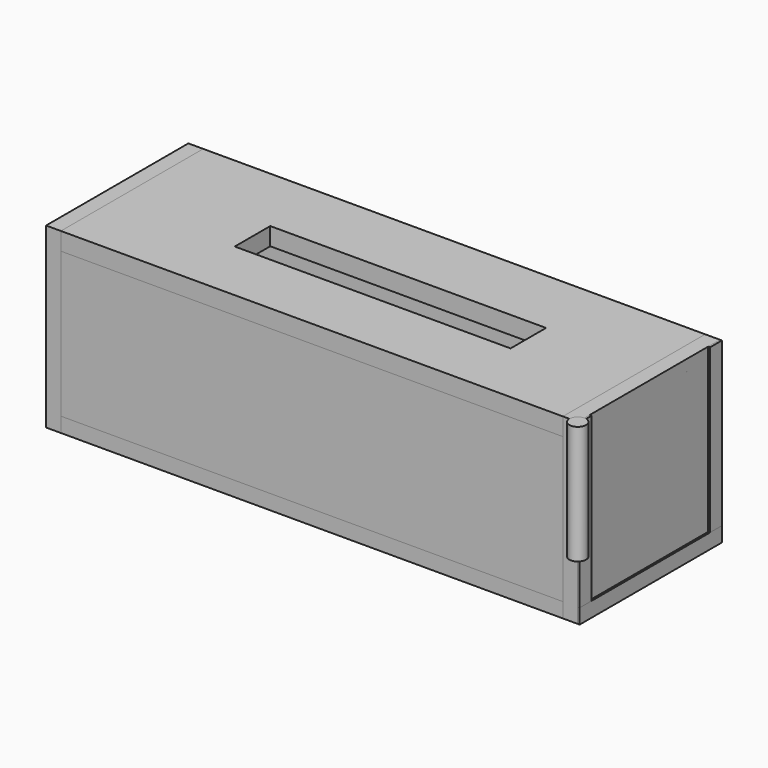
from build123d import *

# Parameters (mm, degrees)
F0_W      = 114.3
F0_H      = 38.1
F1_DEPTH  = 3.175
F2_W      = 114.3
F2_H      = 34.925
F3_DEPTH  = 3.175
F8_W      = 113.8879880309
F8_H      = 3.175
F9_DEPTH  = 3.81
F10_W     = 38.1
F10_H     = 38.1
F11_DEPTH = 3.175
F12_W     = 38.0842164159
F12_H     = 38.1
F13_DEPTH = 3.175
F8_W_2    = 59.0841079511
F8_H_2    = 4.218410936
F8_H_3    = 5.2788990989
F14_DEPTH = 3.175
F15_R     = 1.7975926973
F16_DEPTH = 25.4


# Not quite as in the source:
# - a length typed as a fraction of an inch, garbled in the dataset ("3 / 203.2 mm" for 3/8 in), is restored


with BuildPart() as f1:
    # F0 (on Top) → F1 (new body)
    with BuildSketch(Plane.XY):
        with Locations((57.15, 19.05)):
            Rectangle(F0_W, F0_H)
    extrude(amount=F1_DEPTH)

    # F8 (on face) → F14 (cut)
    with BuildSketch(Plane.XY.offset(38.1)):
        with Locations((58.9459340554, 21.159205468)):
            Rectangle(F8_W_2, F8_H_2)
        with Locations((58.9459340554, 16.4105504505)):
            Rectangle(F8_W_2, F8_H_3)
    extrude(amount=-F14_DEPTH, mode=Mode.SUBTRACT)


with BuildPart() as f3:
    # F2 (on face) → F3 (new body)
    with BuildSketch(Plane.XZ):
        with Locations((57.15, 20.6375)):
            Rectangle(F2_W, F2_H)
    extrude(amount=-F3_DEPTH)


with BuildPart() as f7_1:
    # F7: instance of F3
    add(f3.part.mirror(Plane(origin=(57.15, 19.05, 3.175), x_dir=(1, 0, 0), z_dir=(0, -1, 0))))


with BuildPart() as f9:
    # F8 (on face) → F9 (new body)
    with BuildSketch(Plane.XY.offset(38.1)):
        Polygon((4.0038800798, 19.05), (0, 19.05), (0, 0), (113.8879880309, 0), (113.8879880309, 19.05), (88.4879880309, 19.05), (88.4879880309, 13.7711009011), (29.4038800798, 13.7711009011), (29.4038800798, 19.05), align=None)
        with Locations((56.9439940155, 36.5125)):
            Rectangle(F8_W, F8_H)
        Polygon((113.8879880309, 34.925), (0, 34.925), (0, 19.05), (4.0038800798, 19.05), (29.4038800798, 19.05), (29.4038800798, 23.268410936), (88.4879880309, 23.268410936), (88.4879880309, 19.05), (113.8879880309, 19.05), align=None)
    extrude(amount=-F9_DEPTH)


with BuildPart() as f11:
    # F10 (on face) → F11 (new body)
    with BuildSketch(Plane(origin=(0, 0, 0), x_dir=(0, -1, 0), z_dir=(-1, 0, 0))):
        with Locations((-19.05, 19.05)):
            Rectangle(F10_W, F10_H)
    extrude(amount=-F11_DEPTH)


with BuildPart() as f13:
    # F12 (on face) → F13 (new body)
    with BuildSketch(Plane.YZ.offset(113.8879880309)):
        with Locations((19.0421082079, 19.05)):
            Rectangle(F12_W, F12_H)
    extrude(amount=-F13_DEPTH)


with BuildPart() as f16:
    # F15 (on face) → F16 (new body)
    with BuildSketch(Plane.XY.offset(38.1)):
        with Locations((113.8879880309, 0)):
            Circle(F15_R)
    extrude(amount=-F16_DEPTH)


solid = Compound([f1.part, f3.part, f7_1.part, f9.part, f11.part, f13.part, f16.part])
